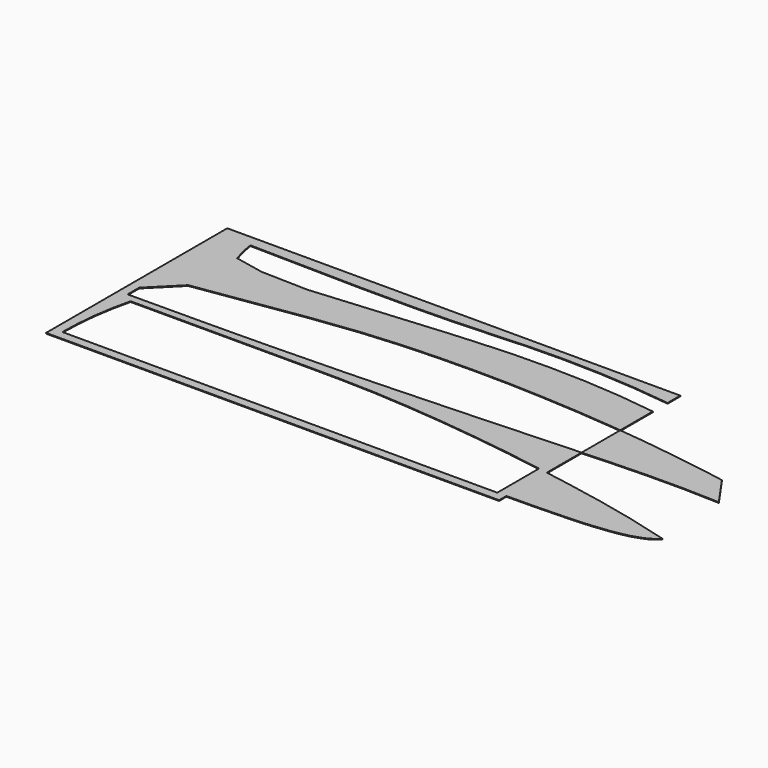
from build123d import *

# Parameters (mm, degrees)
F1_DEPTH = 4


with BuildPart() as f1:
    # F0 (on Top) → F1 (new body)
    with BuildSketch(Plane.XY):
        Polygon((3250, 166), (3050, 219), (3050, 75), (3100, 83), (3150, 94), (3200, 111), (3225, 122), (3250, 137), (3275, 159), align=None)
        Polygon((2500, 329.25), (2500, 50.5), (2650, 52), (2650, 303), align=None)
        Polygon((2650, 303), (2650, 52), (2850, 58), (2850, 264), align=None)
        Polygon((2850, 264), (2850, 58), (2950, 64), (3050, 75), (3050, 219), align=None)
        Polygon((2450, 50), (2500, 50.5), (2500, 329.25), (2450, 338), align=None)
        with BuildLine():
            Line((0, 0), (2500, 0))
            Line((2500, 0), (2500, 50.5))
            Line((2500, 50.5), (2450, 50))
            Line((2450, 50), (2250, 50))
            Line((2250, 50), (2050, 50))
            Line((2050, 50), (1850, 50))
            Line((1850, 50), (1650, 50))
            Line((1650, 50), (1450, 50))
            Line((1450, 50), (1250, 50))
            Line((1250, 50), (1050, 50))
            Line((1050, 50), (50, 50))
            ThreePointArc((50, 50), (62.5465829239, 255.5261540534), (100, 458))
            Line((100, 458), (1050, 458))
            Line((1050, 458), (1250, 457))
            Line((1250, 457), (1450, 451))
            Line((1450, 451), (1650, 438))
            Line((1650, 438), (1850, 420))
            Line((1850, 420), (2050, 397))
            Line((2050, 397), (2250, 370))
            Line((2250, 370), (2450, 338))
            Line((2450, 338), (2500, 329.25))
            Line((2500, 329.25), (2500, 569.25))
            Line((2500, 569.25), (2450, 567))
            Line((2450, 567), (2250, 558))
            Line((2250, 558), (2050, 549))
            Line((2050, 549), (1850, 540))
            Line((1850, 540), (1650, 532))
            Line((1650, 532), (1450, 524))
            Line((1450, 524), (1250, 517))
            Line((1250, 517), (1050, 512))
            Line((1050, 512), (850, 507))
            Line((850, 507), (650, 504))
            Line((650, 504), (450, 502))
            Line((450, 502), (50, 500))
            Line((50, 500), (50, 580))
            Line((50, 580), (200, 730))
            Line((200, 730), (305.4945054945, 746))
            Line((305.4945054945, 746), (800, 821))
            Line((800, 821), (1050, 852))
            Line((1050, 852), (1250, 868))
            Line((1250, 868), (1450, 877))
            Line((1450, 877), (1650, 880))
            Line((1650, 880), (1850, 878))
            Line((1850, 878), (2050, 870))
            Line((2050, 870), (2250, 858))
            Line((2250, 858), (2450, 841))
            Line((2450, 841), (2500, 835.5))
            Line((2500, 835.5), (2500, 1060.2035867911))
            Line((2500, 1060.2035867911), (2495.1732532795, 1061))
            Line((2495.1732532795, 1061), (2295.1732532795, 1085))
            Line((2295.1732532795, 1085), (2095.1732532795, 1099))
            Line((2095.1732532795, 1099), (1895.1732532795, 1104))
            Line((1895.1732532795, 1104), (1695.1732532795, 1101))
            Line((1695.1732532795, 1101), (1495.1732532795, 1090))
            Line((1495.1732532795, 1090), (1355.1732532795, 1080))
            Line((1355.1732532795, 1080), (628.1732532795, 1018))
            Line((628.1732532795, 1018), (370.1732532795, 1025))
            Line((370.1732532795, 1025), (208.1732532795, 1058))
            add(Edge.make_bspline(
                [(177.1732532795, 1188), (182.8605817373, 1144.2682824135), (194.4515766318, 1100.6735346317), (208.1732532795, 1058)],
                knots=[0, 0, 0, 0, 133.645052284, 133.645052284, 133.645052284, 133.645052284], degree=3))
            Line((177.1732532795, 1188), (797.1732532795, 1177))
            Line((797.1732532795, 1177), (1095.1732532795, 1177))
            Line((1095.1732532795, 1177), (1295.1732532795, 1181))
            Line((1295.1732532795, 1181), (1495.1732532795, 1190))
            Line((1495.1732532795, 1190), (1695.1732532795, 1200))
            Line((1695.1732532795, 1200), (1895.1732532795, 1203))
            Line((1895.1732532795, 1203), (2095.1732532795, 1198))
            Line((2095.1732532795, 1198), (2295.1732532795, 1185))
            Line((2295.1732532795, 1185), (2495.1732532795, 1163))
            Line((2495.1732532795, 1163), (2500, 1162.2518542583))
            Line((2500, 1162.2518542583), (2500, 1250))
            Line((2500, 1250), (0, 1250))
            Line((0, 1250), (0, 0))
        make_face()
    extrude(amount=F1_DEPTH)


with BuildPart() as f1b:
    # F0 (on Top) → F1, piece 2 (new body)
    with BuildSketch(Plane.XY):
        Polygon((2500, 835.5), (2500, 569.25), (2650, 576), (2850, 582), (3050, 583), (3251, 577), (3133, 746), (3050, 761), (2850, 792), (2650, 819), align=None)
    extrude(amount=F1_DEPTH)


solid = Compound([f1.part, f1b.part])
